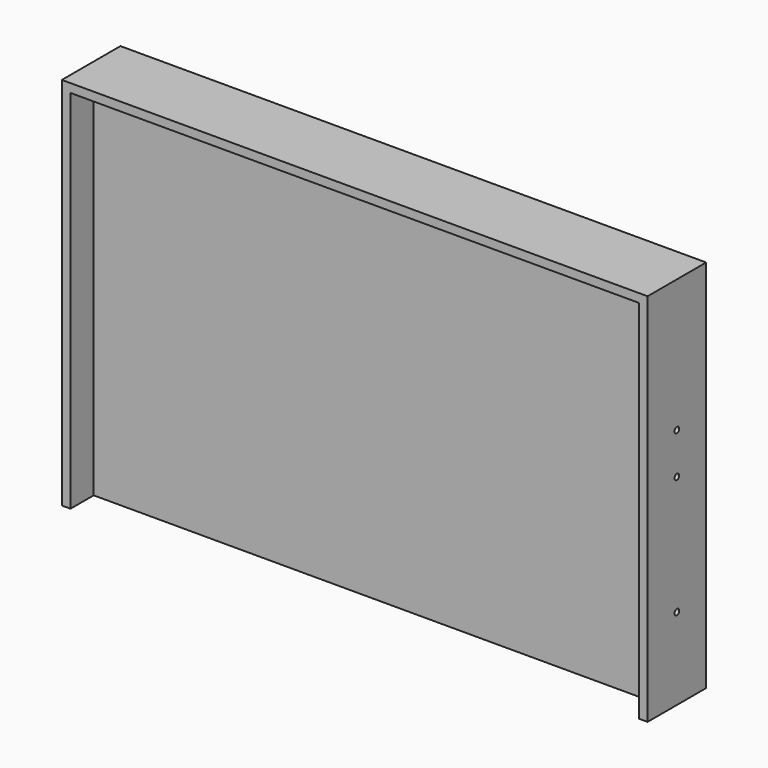
from build123d import *

# Parameters (mm, degrees)
F0_W     = 812.8
F0_H     = 101.6
F1_DEPTH = 12
F3_DEPTH = 508
F4_R     = 3.96875
F5_DEPTH = 9.525
F6_R     = 3.96875
F7_DEPTH = 9.525


# Not quite as in the source:
# - a length typed as a fraction of an inch, garbled in the dataset ("3 / 203.2 mm" for 3/8 in), is restored


with BuildPart() as f1:
    # F0 (on Top) → F1 (new body)
    with BuildSketch(Plane.XY):
        with Locations((406.4, 50.8)):
            Rectangle(F0_W, F0_H)
    extrude(amount=F1_DEPTH)

    # F2 (on face) → F3 (join)
    with BuildSketch(Plane(origin=(0, 0, 0), x_dir=(1, 0, 0), z_dir=(0, 0, -1))):
        Polygon((12, 0), (0, 0), (0, -101.6), (12, -101.6), (12, -52.2239353538), (800.8, -52.2239353538), (800.8, -101.6), (812.8, -101.6), (812.8, 0), (800.8, 0), (800.8, -40.2239353538), (12, -40.2239353538), align=None)
    extrude(amount=F3_DEPTH)

    # F4 (on face) → F5 (cut)
    with BuildSketch(Plane.YZ.offset(812.8)):
        with Locations((50.8, -172.15)):
            Circle(F4_R)
        with Locations((50.8, -229.3)):
            Circle(F4_R)
        with Locations((50.8, -394.4)):
            Circle(F4_R)
    extrude(amount=-F5_DEPTH, mode=Mode.SUBTRACT)

    # F6 (on face) → F7 (cut)
    with BuildSketch(Plane(origin=(0, 0, 0), x_dir=(0, -1, 0), z_dir=(-1, 0, 0))):
        with Locations((-50.8, -172.15)):
            Circle(F6_R)
        with Locations((-50.8, -229.3)):
            Circle(F6_R)
        with Locations((-50.8, -394.4)):
            Circle(F6_R)
    extrude(amount=-F7_DEPTH, mode=Mode.SUBTRACT)


solid = f1.part
